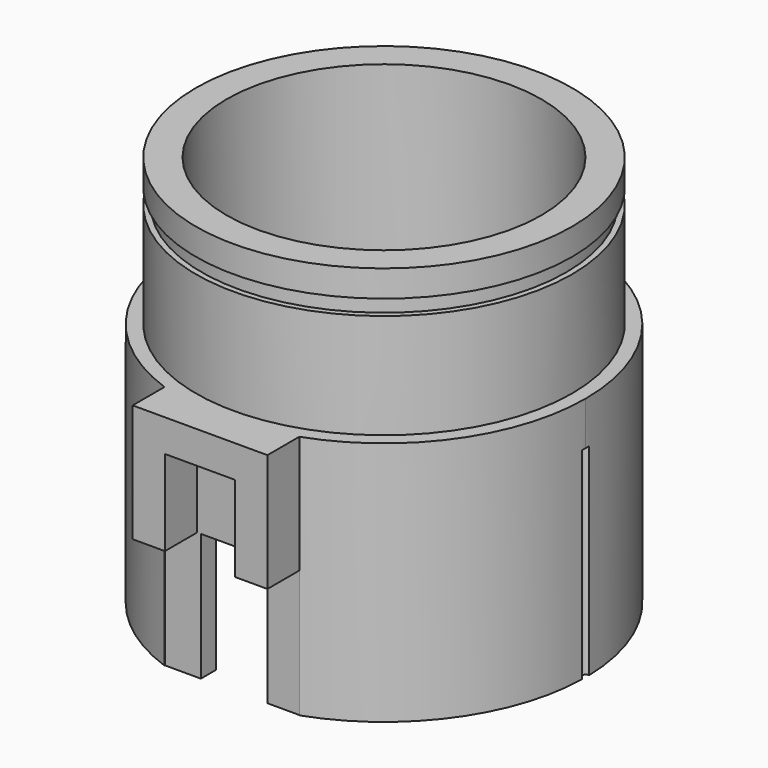
from build123d import *

# Parameters (mm, degrees)
F1_DEPTH      = 7.7216
F2_W          = 2.2098
F2_H          = 4.0132
F2_W_2        = 1.016
F2_H_2        = 2.6924
F3_DEPTH      = 1.27
F5_DEPTH      = 6.35
F6_R          = 5.9182
F6_R_2        = 4.953
F7_DEPTH      = 4.6228
F7_DEPTH_BACK = 2.54
F9_START      = -0.8382
F8_R          = 5.9182
F8_R_2        = 5.7404
F8_R_3        = 4.953
F9_DEPTH      = 0.4826
F11_W         = 2.0946894925
F11_H         = 4.0132
F12_DEPTH     = 0.6219426901


# Not quite as in the source:
# - a fillet or chamfer that OpenCascade refuses, or shapes differently, is made with other operations: its cross-section is extruded or revolved along the edge and cut away or added


with BuildPart() as f1:
    # F0 (on Top) → F1 (new body)
    with BuildSketch(Plane.XY):
        with BuildLine():
            ThreePointArc((2.1209, -5.9853390205), (0, -6.35), (-2.1209, -5.9853390205))
            Line((-2.1209, -5.9853390205), (-2.1209, -7.239))
            Line((-2.1209, -7.239), (2.1209, -7.239))
            Line((2.1209, -7.239), (2.1209, -5.9853390205))
        make_face()
        with BuildLine():
            Line((-2.1209, -5.461), (-2.1209, -5.9853390205))
            ThreePointArc((-2.1209, -5.9853390205), (0, -6.35), (2.1209, -5.9853390205))
            Line((2.1209, -5.9853390205), (2.1209, -5.461))
            Line((2.1209, -5.461), (0, -5.461))
            Line((0, -5.461), (-2.1209, -5.461))
        make_face()
        with BuildLine():
            ThreePointArc((2.1209, -5.9853390205), (5.1860493152, -3.6643406637), (6.35, 0))
            ThreePointArc((6.35, 0), (-3.6643406637, 5.1860493152), (-2.1209, -5.9853390205))
            Line((-2.1209, -5.9853390205), (-2.1209, -5.461))
            Line((-2.1209, -5.461), (0, -5.461))
            Line((0, -5.461), (2.1209, -5.461))
            Line((2.1209, -5.461), (2.1209, -5.9853390205))
        make_face()
        with BuildLine():
            ThreePointArc((5.461, 0), (3.8615101321, -3.8615101321), (0, -5.461))
            ThreePointArc((0, -5.461), (-3.8615101321, 3.8615101321), (5.461, 0))
        make_face(mode=Mode.SUBTRACT)
    extrude(amount=F1_DEPTH)

    # F2 (on face) → F3 (cut)
    with BuildSketch(Plane.XZ.offset(7.239)):
        with Locations((0, 2.0066)):
            Rectangle(F2_W, F2_H)
        with Locations((-1.6129, 2.0066)):
            Rectangle(F2_W_2, F2_H)
        with Locations((1.6129, 2.0066)):
            Rectangle(F2_W_2, F2_H)
        with Locations((0, 5.3594)):
            Rectangle(F2_W, F2_H_2)
    extrude(amount=-F3_DEPTH, mode=Mode.SUBTRACT)

    # F4 (on face) → F5 (cut)
    with BuildSketch(Plane(origin=(0, 0, 0), x_dir=(1, 0, 0), z_dir=(0, 0, -1))):
        with BuildLine():
            ThreePointArc((6.3484633, 0.1396915479), (6.2103, 0), (6.3484633, -0.1396915479))
            ThreePointArc((6.3484633, -0.1396915479), (6.35, 0), (6.3484633, 0.1396915479))
        make_face()
        with BuildLine():
            ThreePointArc((6.3484633, 0.1396915479), (6.35, 0), (6.3484633, -0.1396915479))
            ThreePointArc((6.3484633, -0.1396915479), (6.4482380095, -0.0993246369), (6.4897, 0))
            ThreePointArc((6.4897, 0), (6.4482380095, 0.0993246369), (6.3484633, 0.1396915479))
        make_face()
        with BuildLine():
            ThreePointArc((-6.3484633, -0.1396915479), (-6.2506753631, -0.0982380095), (-6.2103, 0))
            ThreePointArc((-6.2103, 0), (-6.2506753631, 0.0982380095), (-6.3484633, 0.1396915479))
            ThreePointArc((-6.3484633, 0.1396915479), (-6.35, 0), (-6.3484633, -0.1396915479))
        make_face()
        with BuildLine():
            ThreePointArc((-6.3484633, -0.1396915479), (-6.35, 0), (-6.3484633, 0.1396915479))
            ThreePointArc((-6.3484633, 0.1396915479), (-6.4897, 0), (-6.3484633, -0.1396915479))
        make_face()
    extrude(amount=-F5_DEPTH, mode=Mode.SUBTRACT)

    # F6 (on face) → F7 (join, two sides)
    with BuildSketch(Plane.XY.offset(7.7216)) as f7_sk:
        Circle(F6_R)
        Circle(F6_R_2, mode=Mode.SUBTRACT)
    extrude(amount=F7_DEPTH)
    extrude(f7_sk.sketch, amount=-F7_DEPTH_BACK)

    # F8 (on face) → F9 (cut)
    with BuildSketch(Plane.XY.offset(12.3444).offset(F9_START)):
        Circle(F8_R)
        Circle(F8_R_2, mode=Mode.SUBTRACT)
        Circle(F8_R_3)
    extrude(amount=-F9_DEPTH, mode=Mode.SUBTRACT)

    # F10: fillet of radius 1.27 on 1 edges, made by hand

    # F10_s1 → F10_t2 (revolve, cut)
    with BuildSketch(Plane.XZ):
        with BuildLine():
            ThreePointArc((5.461, 5.1816), (5.0870774674, 5.6296387337), (4.953, 6.1976))
            Line((4.953, 6.1976), (4.9276, 6.1976))
            Line((4.9276, 6.1976), (4.9276, 5.1816))
            Line((4.9276, 5.1816), (4.953, 5.1562))
            ThreePointArc((4.953, 5.1562), (5.207, 5.1562), (5.44576, 5.16128))
            Line((5.44576, 5.16128), (5.461, 5.1816))
        make_face()
    revolve(axis=Axis((0, 0, 5.1816), (0, 0, 1)), mode=Mode.SUBTRACT)

    # F11 (on face) → F12 (cut, through all)
    with BuildSketch(Plane.XZ.offset(5.969)):
        with Locations((0.0575552538, 2.0066)):
            Rectangle(F11_W, F11_H)
    extrude(amount=-F12_DEPTH, mode=Mode.SUBTRACT)


solid = f1.part
